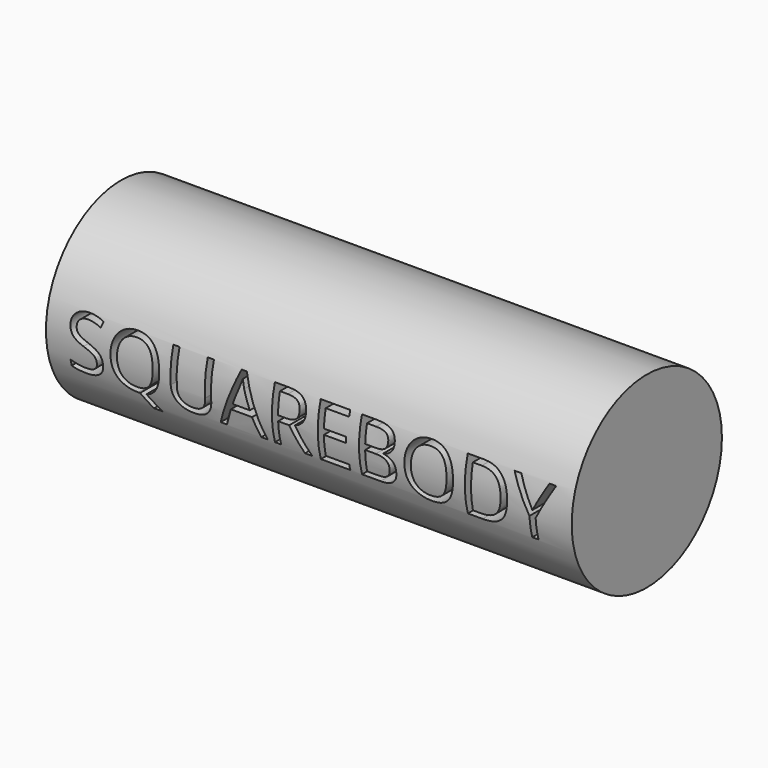
from build123d import *

# Parameters (mm, degrees)
F0_R         = 15.875
F1_DEPTH     = 88.9
F2_TEXT_SIZE = 12.5414363286
F3_DEPTH     = 58.166


# Not quite as in the source:
# - Text() gives the source's letters only with a copy of the font that has no kerning and outlines rounded to 1/6400 em; it was checked with that copy


with BuildPart() as f1:
    # F0 (on Right) → F1 (new body)
    with BuildSketch(Plane.YZ):
        Circle(F0_R)
    extrude(amount=F1_DEPTH)

    # F2 (on Front) → F3 (cut)
    with BuildSketch(Plane.XZ):
        with Locations((3.258813846, -4.5131408588)):
            Text('SQUAREBODY', F2_TEXT_SIZE, font='Open Sans', text_align=(TextAlign.LEFT, TextAlign.BOTTOM))
    extrude(amount=F3_DEPTH, mode=Mode.SUBTRACT)


solid = f1.part
